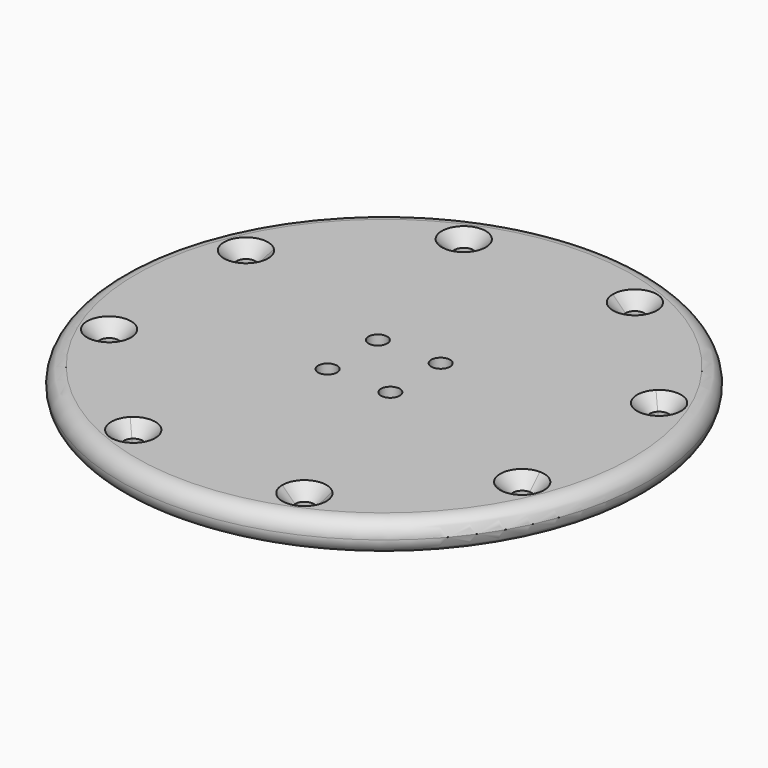
from build123d import *

# Parameters (mm, degrees)
F0_R     = 42
F0_R_2   = 1.5
F1_DEPTH = 5
F2_R     = 2.49999
F3_SIZE  = 2


# Not quite as in the source:
# - a fillet or chamfer is up to 0.001 mm smaller than in the source, because OpenCascade refuses the exact size


with BuildPart() as f1:
    # F0 (on Top) → F1 (new body)
    with BuildSketch(Plane.XY):
        Circle(F0_R)
        with BuildLine():
            ThreePointArc((34.3681841493, 13.6144476452), (33.928844321, 12.5537874734), (32.8681841493, 12.1144476452))
            Line((32.8681841493, 12.1144476452), (32.8681841493, -12.1144476452))
            ThreePointArc((32.8681841493, -12.1144476452), (33.928844321, -12.5537874734), (34.3681841493, -13.6144476452))
            ThreePointArc((34.3681841493, -13.6144476452), (33.4422092978, -15.000266944), (31.8075239775, -14.675107817))
            Line((31.8075239775, -14.675107817), (14.675107817, -31.8075239775))
            ThreePointArc((14.675107817, -31.8075239775), (15.000266944, -32.2941590007), (15.1144476452, -32.8681841493))
            ThreePointArc((15.1144476452, -32.8681841493), (13.6144476452, -34.3681841493), (12.1144476452, -32.8681841493))
            Line((12.1144476452, -32.8681841493), (-12.1144476452, -32.8681841493))
            ThreePointArc((-12.1144476452, -32.8681841493), (-14.1884727937, -34.254003448), (-14.675107817, -31.8075239775))
            Line((-14.675107817, -31.8075239775), (-31.8075239775, -14.675107817))
            ThreePointArc((-31.8075239775, -14.675107817), (-34.254003448, -14.1884727937), (-32.8681841493, -12.1144476452))
            Line((-32.8681841493, -12.1144476452), (-32.8681841493, 12.1144476452))
            ThreePointArc((-32.8681841493, 12.1144476452), (-34.254003448, 14.1884727937), (-31.8075239775, 14.675107817))
            Line((-31.8075239775, 14.675107817), (-14.675107817, 31.8075239775))
            ThreePointArc((-14.675107817, 31.8075239775), (-14.1884727937, 34.254003448), (-12.1144476452, 32.8681841493))
            Line((-12.1144476452, 32.8681841493), (12.1144476452, 32.8681841493))
            ThreePointArc((12.1144476452, 32.8681841493), (13.6144476452, 34.3681841493), (15.1144476452, 32.8681841493))
            ThreePointArc((15.1144476452, 32.8681841493), (15.000266944, 32.2941590007), (14.675107817, 31.8075239775))
            Line((14.675107817, 31.8075239775), (31.8075239775, 14.675107817))
            ThreePointArc((31.8075239775, 14.675107817), (33.4422092978, 15.000266944), (34.3681841493, 13.6144476452))
        make_face(mode=Mode.SUBTRACT)
        with BuildLine():
            Line((32.8681841493, -12.1144476452), (32.8681841493, 12.1144476452))
            ThreePointArc((32.8681841493, 12.1144476452), (31.4823648505, 13.0404224967), (31.8075239775, 14.675107817))
            Line((31.8075239775, 14.675107817), (14.675107817, 31.8075239775))
            ThreePointArc((14.675107817, 31.8075239775), (13.0404224967, 31.4823648505), (12.1144476452, 32.8681841493))
            Line((12.1144476452, 32.8681841493), (-12.1144476452, 32.8681841493))
            ThreePointArc((-12.1144476452, 32.8681841493), (-13.0404224967, 31.4823648505), (-14.675107817, 31.8075239775))
            Line((-14.675107817, 31.8075239775), (-31.8075239775, 14.675107817))
            ThreePointArc((-31.8075239775, 14.675107817), (-31.4823648505, 14.1884727937), (-31.3681841493, 13.6144476452))
            ThreePointArc((-31.3681841493, 13.6144476452), (-31.8075239775, 12.5537874734), (-32.8681841493, 12.1144476452))
            Line((-32.8681841493, 12.1144476452), (-32.8681841493, -12.1144476452))
            ThreePointArc((-32.8681841493, -12.1144476452), (-31.8075239775, -12.5537874734), (-31.3681841493, -13.6144476452))
            ThreePointArc((-31.3681841493, -13.6144476452), (-31.4823648505, -14.1884727937), (-31.8075239775, -14.675107817))
            Line((-31.8075239775, -14.675107817), (-14.675107817, -31.8075239775))
            ThreePointArc((-14.675107817, -31.8075239775), (-13.0404224967, -31.4823648505), (-12.1144476452, -32.8681841493))
            Line((-12.1144476452, -32.8681841493), (12.1144476452, -32.8681841493))
            ThreePointArc((12.1144476452, -32.8681841493), (13.0404224967, -31.4823648505), (14.675107817, -31.8075239775))
            Line((14.675107817, -31.8075239775), (31.8075239775, -14.675107817))
            ThreePointArc((31.8075239775, -14.675107817), (31.4823648505, -13.0404224967), (32.8681841493, -12.1144476452))
        make_face()
        with Locations((-5, -5)):
            Circle(F0_R_2, mode=Mode.SUBTRACT)
        with Locations((5, -5)):
            Circle(F0_R_2, mode=Mode.SUBTRACT)
        with Locations((-5, 5)):
            Circle(F0_R_2, mode=Mode.SUBTRACT)
        with Locations((5, 5)):
            Circle(F0_R_2, mode=Mode.SUBTRACT)
    extrude(amount=F1_DEPTH)

    # F2 (radius 2.5 in the source; OpenCascade refuses exactly that, so slightly less here)
    f2_edges = [f1.edges().sort_by_distance(p)[0] for p in [
        (42, 0, 2.5),
        (-42, 0, 0),
        (-42, 0, 5),
    ]]
    fillet(f2_edges, radius=F2_R)

    # F3
    f3_edges = [f1.edges().sort_by_distance(p)[0] for p in [
        (-34.368184, 13.614448, 5),
        (-12.553787, 33.928844, 5),
        (15.114448, 32.868184, 5),
        (33.928844, 12.553787, 5),
        (32.868184, -15.114448, 5),
        (-15.114448, -32.868184, 5),
        (12.553787, -33.928844, 5),
        (-34.368184, -13.614448, 5),
        (-6.5, -5, 0),
        (-6.5, 5, 0),
        (3.5, 5, 0),
        (3.5, -5, 0),
    ]]
    chamfer(f3_edges, length=F3_SIZE)


solid = f1.part
